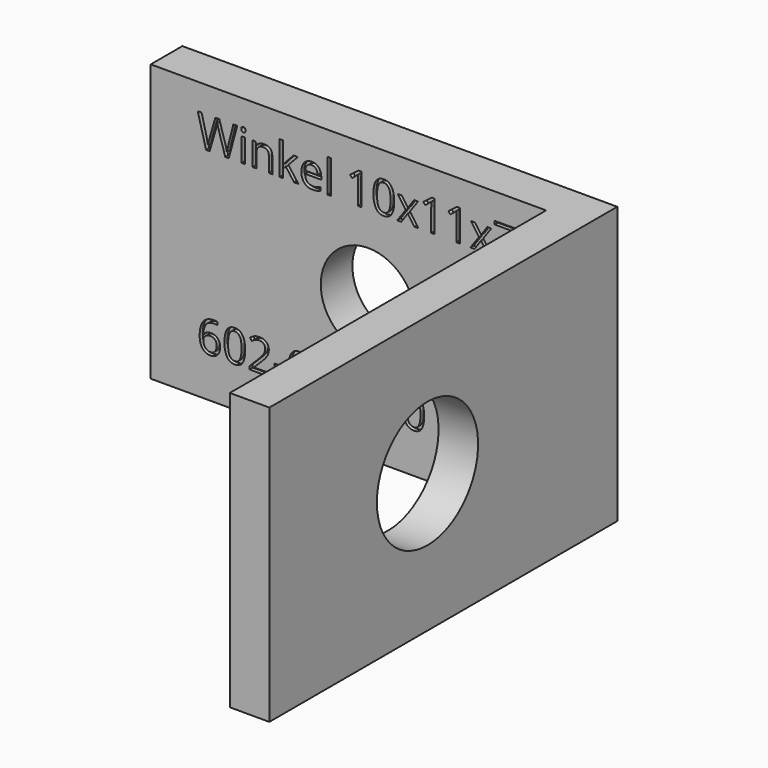
from build123d import *

# Parameters (mm, degrees)
F0_W         = 10
F0_H         = 7
F0_R         = 1.2
F0_W_2       = 1
F1_DEPTH     = 1
F2_DEPTH     = 10
F3_R         = 1.6
F4_DEPTH     = 1
F5_TEXT_SIZE = 1.1111111111
F6_DEPTH     = 0.1


# Not quite as in the source:
# - Text() gives the source's letters only with a copy of the font that has no kerning and outlines rounded to 1/6400 em; it was checked with that copy


with BuildPart() as f1:
    # F0 (on Front) → F1 (new body)
    with BuildSketch(Plane.XZ):
        with Locations((-0.5, 0)):
            Rectangle(F0_W, F0_H)
        Circle(F0_R, mode=Mode.SUBTRACT)
        with Locations((5, 0)):
            Rectangle(F0_W_2, F0_H)
    extrude(amount=-F1_DEPTH)

    # F0 (on Front) → F2 (join)
    with BuildSketch(Plane.XZ):
        with Locations((5, 0)):
            Rectangle(F0_W_2, F0_H)
    extrude(amount=F2_DEPTH)

    # F3 (on face) → F4 (cut, through all)
    with BuildSketch(Plane(origin=(4.5, 0, 0), x_dir=(0, -1, 0), z_dir=(-1, 0, 0))):
        with Locations((5, 0)):
            Circle(F3_R)
    extrude(amount=-F4_DEPTH, mode=Mode.SUBTRACT)

    # F5 (on face) → F6 (cut)
    with BuildSketch(Plane.XZ):
        with Locations((-4.3260041302, 2.0516517666)):
            Text('Winkel 10x11x7', F5_TEXT_SIZE, font='Open Sans', text_align=(TextAlign.LEFT, TextAlign.BOTTOM))
        with Locations((-4.3260041302, -2.4816815668)):
            Text('602-002-00', F5_TEXT_SIZE, font='Open Sans', text_align=(TextAlign.LEFT, TextAlign.BOTTOM))
    extrude(amount=-F6_DEPTH, mode=Mode.SUBTRACT)


solid = f1.part
